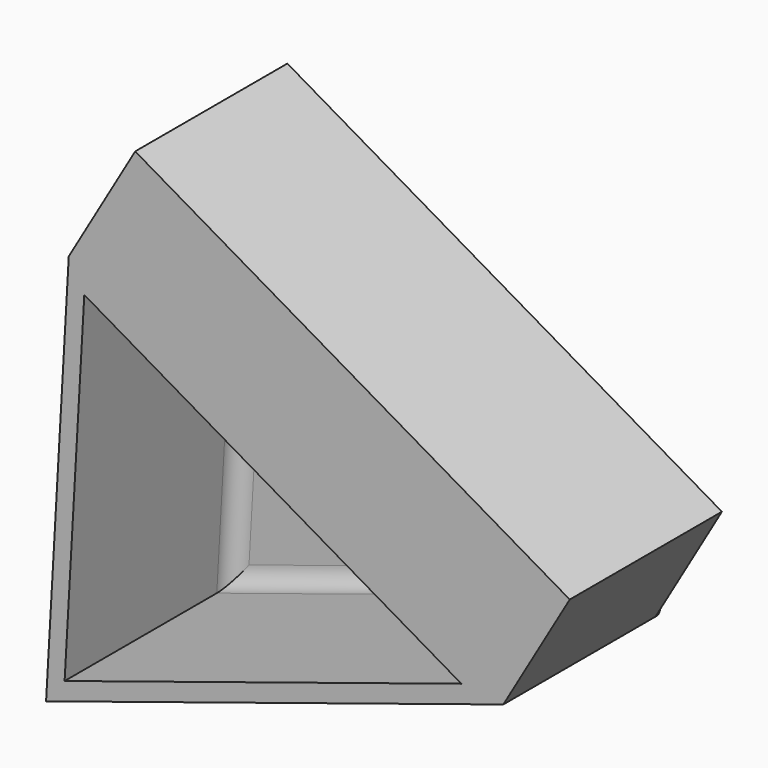
from build123d import *

# Parameters (mm, degrees)
F0_R     = 10.6194281647
F1_DEPTH = 33.274
F3_R     = 5.08
F4_T     = -2.54
F5_DEPTH = 19.558


# Not quite as in the source:
# - the program builds the solid bodies; features that only make, move or delete a surface that nothing else refers to are left out


with BuildPart() as f1:
    # F0 (on Front) → F1 (new body)
    with BuildSketch(Plane.XZ):
        Polygon((0, 17.026649788), (-64.4087642431, 54.5603483915), (-67.7721425891, -4.5970836654), align=None)
        with Locations((-48.2645332813, 22.2235824913)):
            Circle(F0_R, mode=Mode.SUBTRACT)
        with Locations((-48.2645332813, 22.2235824913)):
            Circle(F0_R)
    extrude(amount=F1_DEPTH)

    # F3
    f3_edges = [f1.edges().sort_by_distance(p)[0] for p in [
        (-33.886071, 0, 6.214783),
        (-32.204382, 0, 35.793499),
        (-66.090453, 0, 24.981632),
    ]]
    fillet(f3_edges, radius=F3_R)

    # F4
    f4_openings = [f1.faces().sort_by_distance(p)[0] for p in [
        (-44.060302, -33.274, 22.329972),
    ]]
    offset(amount=F4_T, openings=f4_openings)

    # F5 (add): a face of the model
    f5_faces = [f1.faces().sort_by_distance(p)[0] for p in [
        (-32.2043821216, -19.177, 35.7934990898),
    ]]
    extrude(f5_faces, amount=F5_DEPTH)


solid = f1.part
